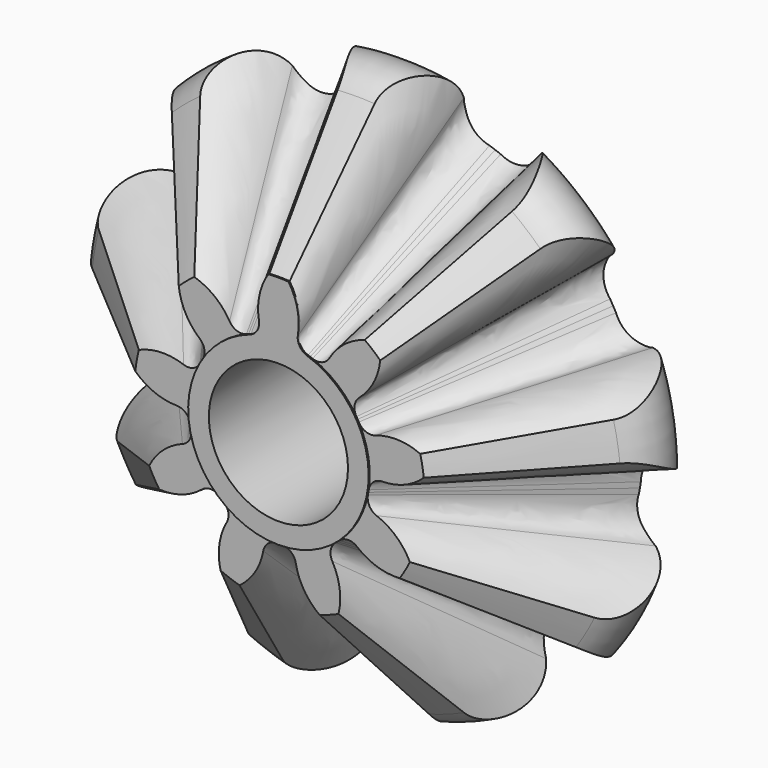
from build123d import *

# Parameters (mm, degrees)
F2_R             = 6.59
F3_DEPTH         = 0.05
F5_DEPTH         = 0.05
F7_DEPTH         = 0.05
F24_COPIES_COUNT = 9
F25_R            = 3.175
F26_R            = 5.08
F27_DEPTH        = 12.7510001


# Not quite as in the source:
# - a pattern or mirror of a feature is missing from the dataset's text; its kind, count and spacing are read off the source's solid


with BuildPart() as f3:
    # F2 (on Front) → F3 (new body, symmetric)
    with BuildSketch(Plane.XZ):
        Circle(F2_R)
    extrude(amount=F3_DEPTH, both=True)

    # F4 (on Front) → F5 (join, symmetric)
    with BuildSketch(Plane.XZ):
        with BuildLine():
            ThreePointArc((-1.1776872799, 6.4839149185), (0, 6.59), (1.1776872799, 6.4839149185))
            ThreePointArc((1.1776872799, 6.4839149185), (1.4579597768, 8.5777511061), (0.7390671926, 10.5641790824))
            ThreePointArc((0.7390671926, 10.5641790824), (0, 10.59), (-0.7390671926, 10.5641790824))
            ThreePointArc((-0.7390671926, 10.5641790824), (-1.4579597768, 8.5777511061), (-1.1776872799, 6.4839149185))
        make_face()
    extrude(amount=F5_DEPTH, both=True)

    # F6 (on Front) → F7 (join, symmetric)
    with BuildSketch(Plane.XZ):
        with BuildLine():
            ThreePointArc((2.0903855568, 6.2496710492), (1.5501113208, 6.6835104035), (1.4215242077, 7.3643761684))
            Line((1.4215242077, 7.3643761684), (-1.4215242077, 7.3643761684))
            ThreePointArc((-1.4215242077, 7.3643761684), (-1.5501113208, 6.6835104035), (-2.0903855568, 6.2496710492))
            ThreePointArc((-2.0903855568, 6.2496710492), (0, 6.59), (2.0903855568, 6.2496710492))
        make_face()
    extrude(amount=F7_DEPTH, both=True)

    # F23 (on face) → F24 section 0
    with BuildSketch(Plane(origin=(0, 0.05, 0), x_dir=(-1, 0, 0), z_dir=(0, 1, 0))):
        with BuildLine():
            ThreePointArc((-0.7390671926, 10.5641790824), (-1.3857142859, 9.0294175925), (-1.4215242077, 7.3643761684))
            ThreePointArc((-1.4215242077, 7.3643761684), (-1.5501113208, 6.6835104035), (-2.0903855568, 6.2496710492))
            ThreePointArc((-2.0903855568, 6.2496710492), (-2.1723367466, 6.2216599923), (-2.2539127445, 6.192574371))
            Line((-2.2539127445, 6.192574371), (0, 0))
            Line((0, 0), (2.2539127445, 6.192574371))
            ThreePointArc((2.2539127445, 6.192574371), (2.1723367466, 6.2216599923), (2.0903855568, 6.2496710492))
            ThreePointArc((2.0903855568, 6.2496710492), (1.5501113208, 6.6835104035), (1.4215242077, 7.3643761684))
            ThreePointArc((1.4215242077, 7.3643761684), (1.3857142859, 9.0294175925), (0.7390671926, 10.5641790824))
            ThreePointArc((0.7390671926, 10.5641790824), (0, 10.59), (-0.7390671926, 10.5641790824))
        make_face()
    # F22 (on offset) → F24 section 1
    with BuildSketch(Plane.XZ.offset(-12.7)):
        with BuildLine():
            ThreePointArc((3.5503431795, 18.3929774522), (3.2488716636, 22.5206123027), (1.8479820326, 26.4149367339))
            ThreePointArc((1.8479820326, 26.4149367339), (0, 26.4795), (-1.8479820326, 26.4149367339))
            ThreePointArc((-1.8479820326, 26.4149367339), (-3.2488716636, 22.5206123027), (-3.5503431795, 18.3929774522))
            ThreePointArc((-3.5503431795, 18.3929774522), (-3.7544889645, 16.620033345), (-5.2169235296, 15.5971494555))
            ThreePointArc((-5.2169235296, 15.5971494555), (-5.4214470868, 15.5272429534), (-5.6250342872, 15.4546546878))
            Line((-5.6250342872, 15.4546546878), (0, 0))
            Line((0, 0), (5.6250342872, 15.4546546878))
            ThreePointArc((5.6250342872, 15.4546546878), (5.4214470868, 15.5272429534), (5.2169235296, 15.5971494555))
            ThreePointArc((5.2169235296, 15.5971494555), (3.7544889645, 16.620033345), (3.5503431795, 18.3929774522))
        make_face()
    f24 = loft()

    # F24_copies: F24 ×9 about axis
    f24_copies_axis = Axis((0, 0, 0), (0, 1, 0))
    for i in range(1, F24_COPIES_COUNT):
        add(f24.rotate(f24_copies_axis, i * 360 / F24_COPIES_COUNT))

    # F25
    f25_edges = [f3.edges().sort_by_distance(p)[0] for p in [
        (0, 12.7, 26.4795),
        (-26.077217, 12.7, 4.598117),
        (-22.93192, 12.7, -13.23975),
        (-9.056522, 12.7, -24.882591),
        (9.056522, 12.7, -24.882591),
        (22.93192, 12.7, -13.23975),
        (26.077217, 12.7, 4.598117),
        (17.020695, 12.7, 20.284474),
        (-17.020695, 12.7, 20.284474),
    ]]
    fillet(f25_edges, radius=F25_R)

    # F26 (on face) → F27 (cut, through all)
    with BuildSketch(Plane.XZ.offset(0.05)):
        Circle(F26_R)
    extrude(amount=-F27_DEPTH, mode=Mode.SUBTRACT)


solid = f3.part
